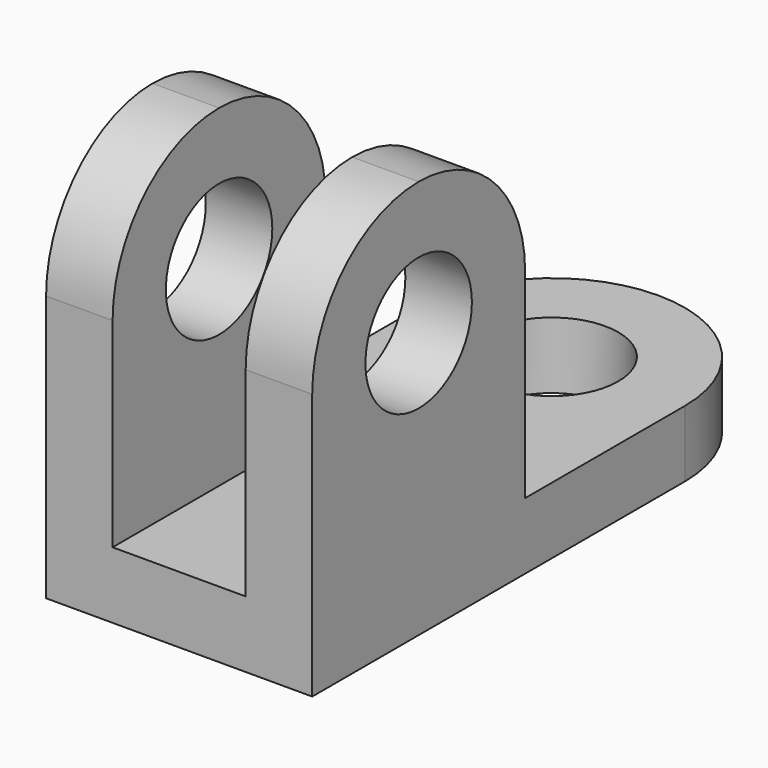
from build123d import *

# Parameters (mm, degrees)
F0_R     = 12.7
F1_DEPTH = 12.7
F2_W     = 12.7
F2_H     = 50.8
F3_DEPTH = 63.5
F4_R     = 25.39999
F6_D     = 25.4


# Not quite as in the source:
# - a fillet or chamfer is up to 0.001 mm smaller than in the source, because OpenCascade refuses the exact size


with BuildPart() as f1:
    # F0 (on Top) → F1 (new body)
    with BuildSketch(Plane.XY):
        with BuildLine():
            Line((0, 88.9), (0, 0))
            Line((0, 0), (50.8, 0))
            Line((50.8, 0), (50.8, 88.9))
            ThreePointArc((50.8, 88.9), (43.3605122421, 106.8605122421), (25.4, 114.3))
            ThreePointArc((25.4, 114.3), (7.4394877579, 106.8605122421), (0, 88.9))
        make_face()
        with Locations((25.4, 88.9)):
            Circle(F0_R, mode=Mode.SUBTRACT)
    extrude(amount=F1_DEPTH)

    # F2 (on face) → F3 (join)
    with BuildSketch(Plane.XY.offset(12.7)):
        with Locations((6.35, 25.4)):
            Rectangle(F2_W, F2_H)
        with Locations((44.45, 25.4)):
            Rectangle(F2_W, F2_H)
    extrude(amount=F3_DEPTH)

    # F4 (radius 25.4 in the source; OpenCascade refuses exactly that, so slightly less here)
    f4_edges = [f1.edges().sort_by_distance(p)[0] for p in [
        (6.35, 50.8, 76.2),
        (6.35, 0, 76.2),
        (44.45, 0, 76.2),
        (44.45, 50.8, 76.2),
    ]]
    fillet(f4_edges, radius=F4_R)

    # F6 (through all)
    with Locations(Plane(origin=(0, 0, 0), x_dir=(0, -1, 0), z_dir=(-1, 0, 0))):
        with Locations((-25.4, 50.8)):
            Hole(F6_D / 2)


solid = f1.part
